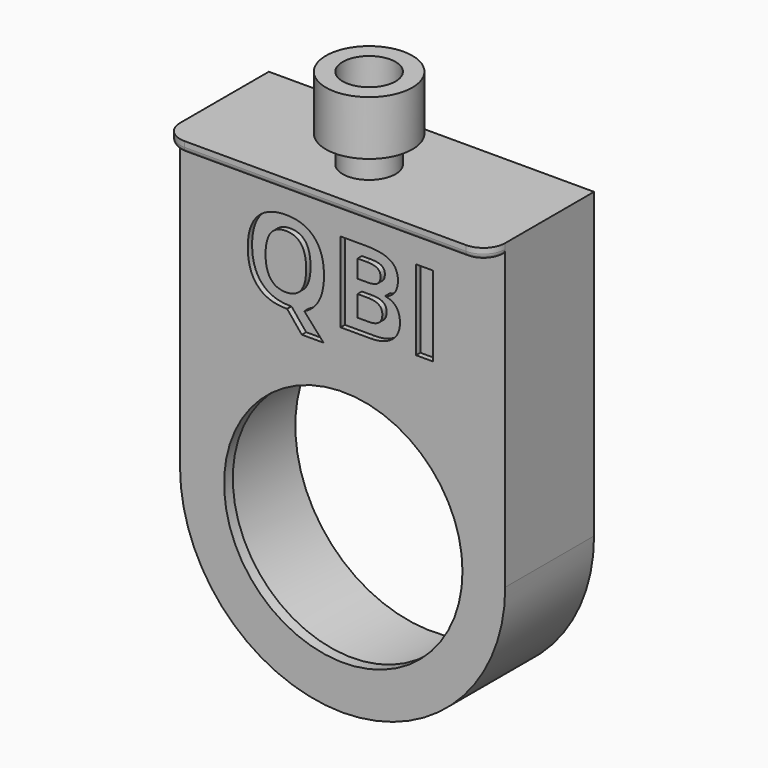
from build123d import *

# Parameters (mm, degrees)
F0_R         = 12.569468159
F1_DEPTH     = 10.2
F2_R         = 12.569468159
F2_R_2       = 10.9516753933
F3_DEPTH     = 1
F5_DEPTH     = 1
F6_R         = 0.5
F7_TEXT_SIZE = 10.3037396912
F8_DEPTH     = 0.5
F9_R         = 2.428504216
F10_DEPTH    = 5
F11_R        = 3.9689267518
F11_R_2      = 2.428504216
F12_DEPTH    = 2.5


# Not quite as in the source:
# - Text() gives the source's letters only with a copy of the font that has no kerning and outlines rounded to 1/6400 em; it was checked with that copy


with BuildPart() as f1:
    # F0 (on Front) → F1 (new body)
    with BuildSketch(Plane.XZ):
        with BuildLine():
            Line((9.2994272709, -18.6363415956), (9.2994272709, 9.1973861888))
            Line((9.2994272709, 9.1973861888), (-20.5795679033, 9.1973861888))
            Line((-20.5795679033, 9.1973861888), (-20.5795679033, -18.6363415956))
            ThreePointArc((-20.5795679033, -18.6363415956), (-16.2075389277, -29.2215308667), (-5.6400703162, -33.6362195771))
            ThreePointArc((-5.6400703162, -33.6362195771), (4.9273982954, -29.2215308667), (9.2994272709, -18.6363415956))
        make_face()
        with Locations((-5.5795679033, -18.6363415956)):
            Circle(F0_R, mode=Mode.SUBTRACT)
    extrude(amount=F1_DEPTH)

    # F2 (on face) → F3 (join)
    with BuildSketch(Plane.XZ.offset(10.2)):
        with Locations((-5.5795679033, -18.6363415956)):
            Circle(F2_R)
        with Locations((-5.5795679033, -18.6363415956)):
            Circle(F2_R_2, mode=Mode.SUBTRACT)
    extrude(amount=-F3_DEPTH)

    # F4 (on face) → F5 (join)
    with BuildSketch(Plane.XY.offset(9.1973861888)):
        with BuildLine():
            Line((9.2994272709, -10.2), (-20.5795679033, -10.2))
            ThreePointArc((-20.5795679033, -10.2), (-19.9937814657, -11.6142135624), (-18.5795679033, -12.2))
            Line((-18.5795679033, -12.2), (7.2994272709, -12.2))
            ThreePointArc((7.2994272709, -12.2), (8.7136408333, -11.6142135624), (9.2994272709, -10.2))
        make_face()
    extrude(amount=-F5_DEPTH)

    # F6
    f6_edges = [f1.edges().sort_by_distance(p)[0] for p in [
        (-5.64007, -12.2, 8.197386),
        (-19.993781, -11.614214, 8.197386),
        (8.713641, -11.614214, 8.197386),
    ]]
    fillet(f6_edges, radius=F6_R)

    # F7 (on face) → F8 (cut, symmetric)
    with BuildSketch(Plane.XZ.offset(10.2)):
        with Locations((-14.9547662586, -2.5381632149)):
            Text('QBI', F7_TEXT_SIZE, font='Open Sans', font_style=FontStyle.BOLD, text_align=(TextAlign.LEFT, TextAlign.BOTTOM))
    extrude(amount=F8_DEPTH, both=True, mode=Mode.SUBTRACT)

    # F9 (on face) → F10 (join)
    with BuildSketch(Plane.XY.offset(9.1973861888)):
        with Locations((-5.9675336815, -6.7469635978)):
            Circle(F9_R)
    extrude(amount=F10_DEPTH)

    # F11 (on face) → F12 (join, symmetric)
    with BuildSketch(Plane.XY.offset(14.1973861888)):
        with Locations((-5.9675336815, -6.7469635978)):
            Circle(F11_R)
        with Locations((-5.9675336815, -6.7469635978)):
            Circle(F11_R_2, mode=Mode.SUBTRACT)
    extrude(amount=F12_DEPTH, both=True)


solid = f1.part
